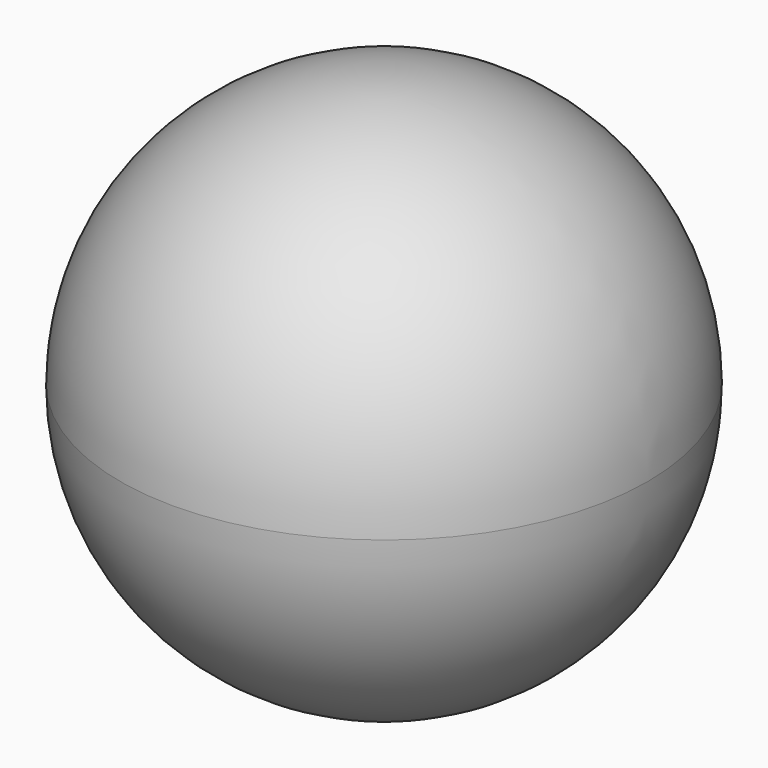
from build123d import *


with BuildPart() as f1:
    # F0 (on Front) → F1 (revolve)
    with BuildSketch(Plane.XZ):
        with BuildLine():
            ThreePointArc((0, -8), (5.6568542495, -5.6568542495), (8, 0))
            ThreePointArc((8, 0), (5.6568542495, 5.6568542495), (0, 8))
            Line((0, 8), (0, 0))
            Line((0, 0), (0, -8))
        make_face()
    revolve(axis=Axis((0, 0, 10.4239946231), (0, 0, 1)))


solid = f1.part
